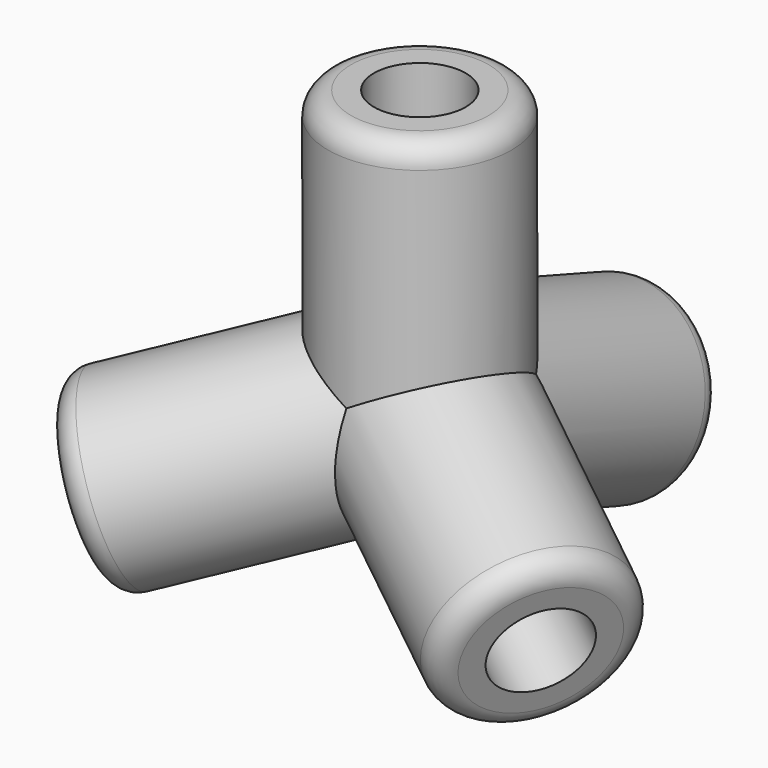
from build123d import *

# Parameters (mm, degrees)
F0_R      = 2
F1_DEPTH  = 6
F4_R      = 2
F5_DEPTH  = 6
F6_R      = 1
F9_DEPTH  = 4
F8_R      = 1
F10_DEPTH = 4
F11_COUNT = 3
F12_R     = 0.5


with BuildPart() as f1:
    # F0 (on Top) → F1 (new body)
    with BuildSketch(Plane.XY):
        Circle(F0_R)
    extrude(amount=F1_DEPTH)

    # F4 (on line) → F5 (join)
    with BuildSketch(Plane(origin=(0, 0, 0), x_dir=(1, 0, 0), z_dir=(0, -0.9426414911, 0.3338068592))):
        Circle(F4_R)
    extrude(amount=-F5_DEPTH)

    # F6 (on face) → F9 (cut)
    with BuildSketch(Plane.XY.offset(6)):
        Circle(F6_R)
    extrude(amount=-F9_DEPTH, mode=Mode.SUBTRACT)

    # F8 (on face) → F10 (cut)
    with BuildSketch(Plane(origin=(0, 5.6558489466, -2.0028411554), x_dir=(-1, 0, 0), z_dir=(0, 0.9426414911, -0.3338068592))):
        Circle(F8_R)
    extrude(amount=-F10_DEPTH, mode=Mode.SUBTRACT)

    # F11: F1 ×3 about axis
    f11_axis = Axis((0, 0, 23.5362444073), (0, 0, 1))


with BuildPart() as f1_1:
    add(f1.part)
    for i in range(1, F11_COUNT):
        add(f1.part.rotate(f11_axis, i * 360 / F11_COUNT))

    # F12
    f12_edges = [f1_1.edges().sort_by_distance(p)[0] for p in [
        (-2, 0, 6),
        (5.898109, -1.095874, -2.002841),
        (-2, 5.655849, -2.002841),
        (-3.898109, -4.559975, -2.002841),
    ]]
    fillet(f12_edges, radius=F12_R)


solid = f1_1.part
